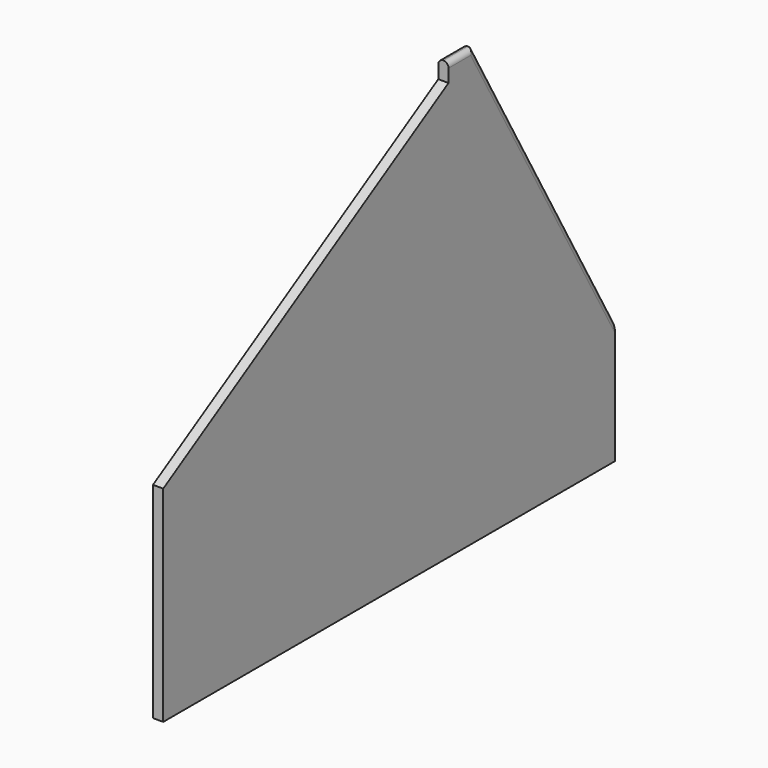
from build123d import *

# Parameters (mm, degrees)
F0_W     = 113.7219756842
F0_H     = 120
F0_W_2   = 107.0308029652
F0_H_2   = 200
F1_DEPTH = 10
F2_R     = 4.99999


# Not quite as in the source:
# - a fillet or chamfer is up to 0.001 mm smaller than in the source, because OpenCascade refuses the exact size


with BuildPart() as f1:
    # F0 (on Right) → F1 (new body)
    with BuildSketch(Plane.YZ):
        with Locations((211.910609901, -14.3104368448)):
            Rectangle(F0_W, F0_H)
        Polygon((95.8531785295, -74.3104368448), (155.0496220589, -74.3104368448), (155.0496220589, 45.6895631552), (268.771597743, 45.6895631552), (95.8531785295, 349.9907631145), align=None)
        Polygon((66.0946071148, -74.3104368448), (95.8531785295, -74.3104368448), (95.8531785295, 349.9907631145), (66.0946071148, 332.2893329267), align=None)
        Polygon((66.0946071148, 332.2893329267), (95.8531785295, 349.9907631145), (66.0946071148, 349.9907631145), align=None)
        Polygon((-174.1975992918, -74.3104368448), (66.0946071148, -74.3104368448), (66.0946071148, 332.2893329267), (-281.228402257, 125.6895631552), (-174.1975992918, 125.6895631552), align=None)
        with Locations((-227.7130007744, 25.6895631552)):
            Rectangle(F0_W_2, F0_H_2)
    extrude(amount=F1_DEPTH)

    # F2 (radius 5 in the source; OpenCascade refuses exactly that, so slightly less here)
    f2_edges = [f1.edges().sort_by_distance(p)[0] for p in [
        (10, 182.312388, 197.840163),
        (0, 182.312388, 197.840163),
        (10, 80.973893, 349.990763),
        (0, 80.973893, 349.990763),
    ]]
    fillet(f2_edges, radius=F2_R)


solid = f1.part
